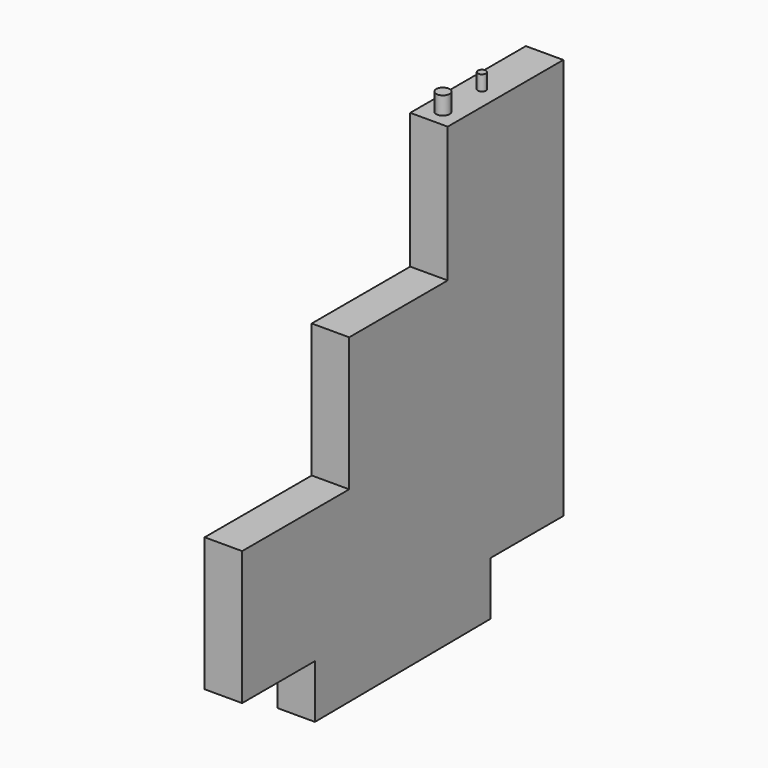
from build123d import *

# Parameters (mm, degrees)
F1_DEPTH = 7
F2_R     = 1.25
F3_DEPTH = 25
F2_R_2   = 0.75
F4_DEPTH = 25
F5_DEPTH = 66
F6_DEPTH = 65.5


# Not quite as in the source:
# - a feature names something its author has since deleted; it is built from what else it names


with BuildPart() as f1:
    # F0 (on Right) → F1 (new body)
    with BuildSketch(Plane.YZ):
        Polygon((-25.6658861851, 12.3832505633), (-25.6658861851, -12.6167494367), (-8.6658861851, -12.6167494367), (-8.6658861851, -22.6167494367), (32.3341138149, -22.3259466936), (32.3341138149, -12.3259466936), (49.3341138149, -12.3259466936), (49.3341138149, 62.6740533064), (26.7576448203, 62.6740533064), (22.3341138149, 62.6740533064), (22.3341138149, 37.3832505633), (-0.6658861851, 37.3832505633), (-0.6658861851, 12.3832505633), align=None)
    extrude(amount=F1_DEPTH)



with BuildPart() as f3:
    # F2 (on Top) → F3 (new body)
    with BuildSketch(Plane.XY):
        with Locations((3.5, 25.5862374604)):
            Circle(F2_R)
    extrude(amount=F3_DEPTH)

    # F2 (on Top) → F4 (join)
    with BuildSketch(Plane.XY):
        with Locations((3.5, 25.5862374604)):
            Circle(F2_R)
    extrude(amount=F4_DEPTH)


with BuildPart() as f3b:
    # F2 (on Top) → F3, piece 2 (new body)
    with BuildSketch(Plane.XY):
        with Locations((3.5, 34.6862374604)):
            Circle(F2_R_2)
    extrude(amount=F3_DEPTH)

    # F2 (on Top) → F4, piece 2 (join)
    with BuildSketch(Plane.XY):
        with Locations((3.5, 34.6862374604)):
            Circle(F2_R_2)
    extrude(amount=F4_DEPTH)


with BuildPart() as f1_1:
    add(f1.part)

    add(f3.part)  # F5 merges F3
    # F2 (on Top) → F5 (join)
    with BuildSketch(Plane.XY):
        with Locations((3.5, 25.5862374604)):
            Circle(F2_R)
    extrude(amount=F5_DEPTH)


    add(f3b.part)  # F6 merges F3b
    # F2 (on Top) → F6 (join)
    with BuildSketch(Plane.XY):
        with Locations((3.5, 34.6862374604)):
            Circle(F2_R_2)
    extrude(amount=F6_DEPTH)


solid = f1_1.part
